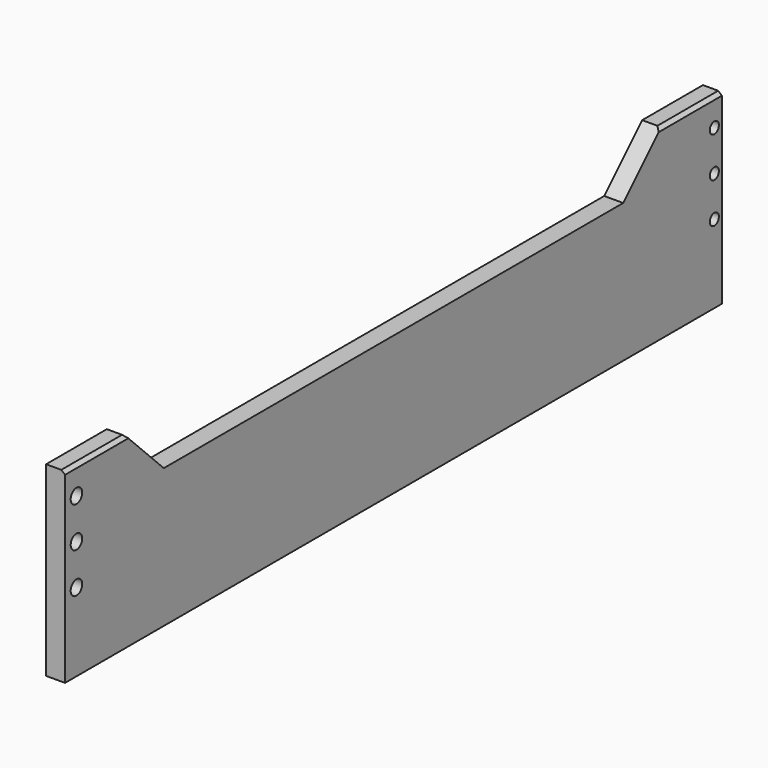
from build123d import *

# Parameters (mm, degrees)
F1_DEPTH = 6.35
F2_D     = 4.826
F3_D     = 3.81
F4_SIZE2 = 6.3416783923
F4_SIZE  = 5.3213
F6_DEPTH = 25.4


# Not quite as in the source:
# - a feature names something its author has since deleted; it is built from what else it names


with BuildPart() as f1:
    # F0 (on Right) → F1 (new body)
    with BuildSketch(Plane.YZ):
        Polygon((274.6375, -12.7), (274.6375, 0), (274.6375, 53.8988), (0, 53.8988), (0, 0), (0, -12.7), align=None)
    extrude(amount=F1_DEPTH)

    # F2 (through all)
    with Locations(Plane(origin=(0, 0, 0), x_dir=(0, 1, 0), z_dir=(-1, 0, 0))):
        with Locations((4.7625, -40.4241), (4.7625, -26.9494), (4.7625, -13.4747)):
            Hole(F2_D / 2)

    # F3 (through all)
    with Locations(Plane(origin=(0, 0, 0), x_dir=(0, 1, 0), z_dir=(-1, 0, 0))):
        with Locations((271.4625, -40.4241), (271.4625, -26.9494), (271.4625, -13.4747)):
            Hole(F3_D / 2)

    # F4
    f4_edges = [f1.edges().sort_by_distance(p)[0] for p in [
        (6.35, 137.31875, 53.8988),
    ]]
    f4_side = f1.faces().sort_by_distance((6.35, 137.466328, 20.568323))[0]
    chamfer(f4_edges, length=F4_SIZE, length2=F4_SIZE2, reference=f4_side)

    # F5 (on face) → F6 (cut)
    with BuildSketch(Plane(origin=(0, 0, 0), x_dir=(0, -1, 0), z_dir=(-1, 0, 0))):
        Polygon((-274.6375, 53.8988), (-274.6375, 49.6316), (-249.2375, 49.6316), (-233.3625, 33.7566), (-41.275, 33.7566), (-25.4, 49.6316), (0, 49.6316), (0, 53.8988), align=None)
    extrude(amount=-F6_DEPTH, mode=Mode.SUBTRACT)


solid = f1.part
